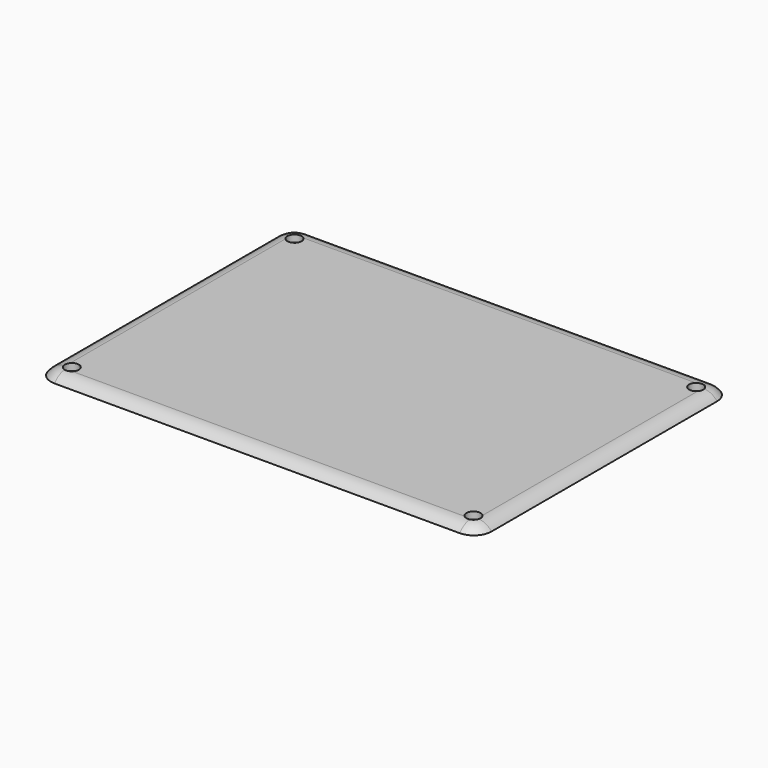
from build123d import *

# Parameters (mm, degrees)
F1_DEPTH     = 2
F0_W         = 2
F0_H         = 68
F0_W_2       = 103
F0_H_2       = 2
F2_DEPTH     = 2
F3_R         = 2
F4_DEPTH     = 5
F5_R         = 5
F6_T1_DEPTH  = 80
F6_T3_DEPTH  = 115
F6_T6_ANGLE  = 90
F6_T8_ANGLE  = 90
F6_T10_ANGLE = 90
F6_T12_ANGLE = 90


# Not quite as in the source:
# - a fillet or chamfer that OpenCascade refuses, or shapes differently, is made with other operations: its cross-section is extruded or revolved along the edge and cut away or added


with BuildPart() as f1:
    # F0 (on Top) → F1 (new body)
    with BuildSketch(Plane.XY):
        Polygon((-51.5, -43), (51.5, -43), (51.5, -34), (60.5, -34), (60.5, 34), (51.5, 34), (51.5, 43), (-51.5, 43), (-51.5, 34), (-60.5, 34), (-60.5, -34), (-51.5, -34), align=None)
    extrude(amount=F1_DEPTH)

    # F0 (on Top) → F2 (join)
    with BuildSketch(Plane.XY):
        Polygon((-62.5, -45), (-51.5, -45), (-51.5, -43), (-51.5, -34), (-60.5, -34), (-62.5, -34), align=None)
        with Locations((-61.5, 0)):
            Rectangle(F0_W, F0_H)
        with Locations((0, -44)):
            Rectangle(F0_W_2, F0_H_2)
        Polygon((51.5, -45), (62.5, -45), (62.5, -34), (60.5, -34), (51.5, -34), (51.5, -43), align=None)
        with Locations((61.5, 0)):
            Rectangle(F0_W, F0_H)
        Polygon((60.5, 34), (62.5, 34), (62.5, 45), (51.5, 45), (51.5, 43), (51.5, 34), align=None)
        with Locations((0, 44)):
            Rectangle(F0_W_2, F0_H_2)
        Polygon((-62.5, 45), (-62.5, 34), (-60.5, 34), (-51.5, 34), (-51.5, 43), (-51.5, 45), align=None)
    extrude(amount=F2_DEPTH)

    # F3 (on face) → F4 (cut)
    with BuildSketch(Plane.XY.offset(2)):
        with Locations((-57, -39.5)):
            Circle(F3_R)
        with Locations((57, -39.5)):
            Circle(F3_R)
        with Locations((-57, 39.5)):
            Circle(F3_R)
        with Locations((57, 39.5)):
            Circle(F3_R)
    extrude(amount=-F4_DEPTH, mode=Mode.SUBTRACT)

    # F5
    f5_edges = [f1.edges().sort_by_distance(p)[0] for p in [
        (-62.5, 45, 1),
        (62.5, 45, 1),
        (62.5, -45, 1),
        (-62.5, -45, 1),
    ]]
    fillet(f5_edges, radius=F5_R)

    # F6: fillet of radius 5 on 1 edges, made by hand

    # F6_s2 → F6_t1 (cut)
    with BuildSketch(Plane.XZ.offset(-40)):
        with BuildLine():
            ThreePointArc((-62.5, 0), (-60.7360679775, 1.472135955), (-58.5, 2))
            Line((-58.5, 2), (-62.5, 2))
            Line((-62.5, 2), (-62.5, 0))
        make_face()
        with BuildLine():
            ThreePointArc((62.5, 0), (60.7360679775, 1.472135955), (58.5, 2))
            Line((58.5, 2), (62.5, 2))
            Line((62.5, 2), (62.5, 0))
        make_face()
    extrude(amount=F6_T1_DEPTH, mode=Mode.SUBTRACT)

    # F6_s4 → F6_t3 (cut)
    with BuildSketch(Plane.YZ.offset(-57.5)):
        with BuildLine():
            ThreePointArc((-45, 0), (-43.2360679775, 1.472135955), (-41, 2))
            Line((-41, 2), (-45, 2))
            Line((-45, 2), (-45, 0))
        make_face()
        with BuildLine():
            ThreePointArc((45, 0), (43.2360679775, 1.472135955), (41, 2))
            Line((41, 2), (45, 2))
            Line((45, 2), (45, 0))
        make_face()
    extrude(amount=F6_T3_DEPTH, mode=Mode.SUBTRACT)

    # F6_s5 → F6_t6 (revolve, cut)
    with BuildSketch(Plane.XZ.offset(-40)):
        with BuildLine():
            ThreePointArc((-62.5, 0), (-60.7360679775, 1.472135955), (-58.5, 2))
            Line((-58.5, 2), (-62.5, 2))
            Line((-62.5, 2), (-62.5, 0))
        make_face()
    revolve(axis=Axis((-57.5, 40, 2), (0, 0, -1)), revolution_arc=F6_T6_ANGLE, mode=Mode.SUBTRACT)

    # F6_s7 → F6_t8 (revolve, cut)
    with BuildSketch(Plane.YZ.offset(-57.5)):
        with BuildLine():
            ThreePointArc((-45, 0), (-43.2360679775, 1.472135955), (-41, 2))
            Line((-41, 2), (-45, 2))
            Line((-45, 2), (-45, 0))
        make_face()
    revolve(axis=Axis((-57.5, -40, 2), (0, 0, -1)), revolution_arc=F6_T8_ANGLE, mode=Mode.SUBTRACT)

    # F6_s9 → F6_t10 (revolve, cut)
    with BuildSketch(Plane.YZ.offset(57.5)):
        with BuildLine():
            ThreePointArc((-45, 0), (-43.2360679775, 1.472135955), (-41, 2))
            Line((-41, 2), (-45, 2))
            Line((-45, 2), (-45, 0))
        make_face()
    revolve(axis=Axis((57.5, -40, 2), (0, 0, 1)), revolution_arc=F6_T10_ANGLE, mode=Mode.SUBTRACT)

    # F6_s11 → F6_t12 (revolve, cut)
    with BuildSketch(Plane.XZ.offset(-40)):
        with BuildLine():
            ThreePointArc((62.5, 0), (60.7360679775, 1.472135955), (58.5, 2))
            Line((58.5, 2), (62.5, 2))
            Line((62.5, 2), (62.5, 0))
        make_face()
    revolve(axis=Axis((57.5, 40, 2), (0, 0, 1)), revolution_arc=F6_T12_ANGLE, mode=Mode.SUBTRACT)


solid = f1.part
